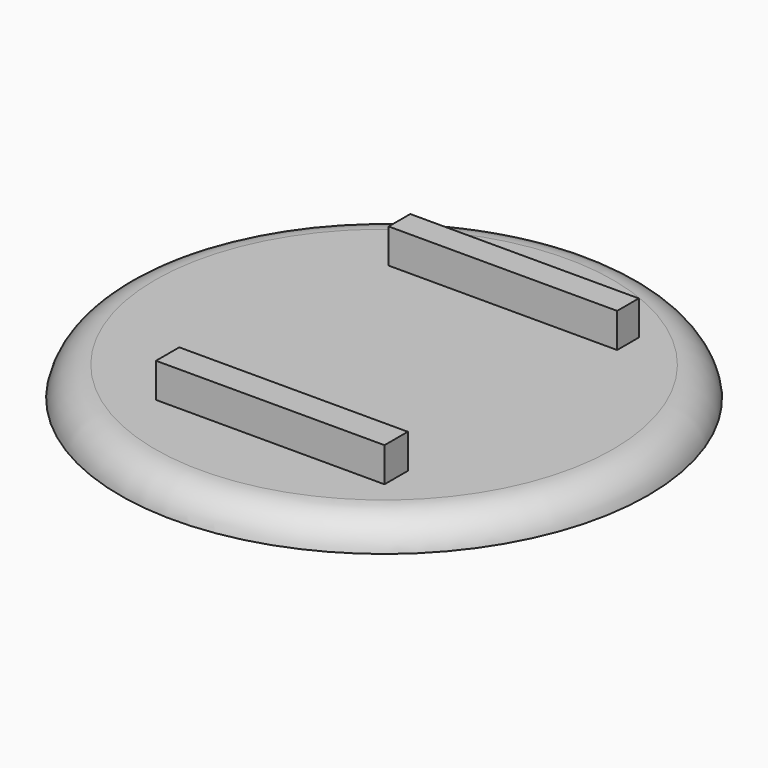
from build123d import *

# Parameters (mm, degrees)
F0_R     = 35.9935602645
F1_DEPTH = 4
F3_W     = 31.1600742862
F3_H     = 3.6825519055
F3_H_2   = 3.9658267051
F4_DEPTH = 4.7
F6_DEPTH = 2


# Not quite as in the source:
# - a fillet or chamfer that OpenCascade refuses, or shapes differently, is made with other operations: its cross-section is extruded or revolved along the edge and cut away or added


with BuildPart() as f1:
    # F0 (on Top) → F1 (new body)
    with BuildSketch(Plane.XY):
        Circle(F0_R)
    extrude(amount=F1_DEPTH)

    # F2: fillet of radius 4.8284271247 on 1 edges, made by hand

    # F2_s1 → F2_t2 (revolve, cut)
    with BuildSketch(Plane.XZ):
        with BuildLine():
            ThreePointArc((35.9935602645, 0), (34.3442797526, 2.8670910053), (31.2367318045, 4))
            Line((31.2367318045, 4), (35.9935602645, 4))
            Line((35.9935602645, 4), (35.9935602645, 0))
        make_face()
    revolve(axis=Axis((0, 0, 4), (0, 0, 1)), mode=Mode.SUBTRACT)

    # F3 (on face) → F4 (join)
    with BuildSketch(Plane.XY.offset(4)):
        with Locations((1.6996399499, 19.9707737193)):
            Rectangle(F3_W, F3_H)
        with Locations((1.6996399499, -19.5458633825)):
            Rectangle(F3_W, F3_H_2)
    extrude(amount=F4_DEPTH)

    # F5 (on face) → F6 (cut)
    with BuildSketch(Plane(origin=(0, 0, 0), x_dir=(1, 0, 0), z_dir=(0, 0, -1))):
        with BuildLine():
            Line((1.0116308873, -10.4608191177), (4.1609390889, -1.4550810977))
            ThreePointArc((4.1609390889, -1.4550810977), (-0.0142907136, -4.4080007801), (-4.1702862527, -1.4280713123))
            Line((-4.1702862527, -1.4280713123), (-1.0771154127, -10.4608191177))
            Line((-1.0771154127, -10.4608191177), (-1.0116308873, -10.4608191177))
            ThreePointArc((-1.0116308873, -10.4608191177), (0, -9.4491882305), (1.0116308873, -10.4608191177))
        make_face()
        with BuildLine():
            ThreePointArc((-1.0116308873, -10.4608191177), (0, -11.472450005), (1.0116308873, -10.4608191177))
            Line((1.0116308873, -10.4608191177), (0, -10.4608191177))
            Line((0, -10.4608191177), (-1.0116308873, -10.4608191177))
        make_face()
        with BuildLine():
            Line((0, -10.4608191177), (1.0116308873, -10.4608191177))
            ThreePointArc((1.0116308873, -10.4608191177), (0, -9.4491882305), (-1.0116308873, -10.4608191177))
            Line((-1.0116308873, -10.4608191177), (0, -10.4608191177))
        make_face()
        with BuildLine():
            ThreePointArc((4.1609390889, -1.4550810977), (4.3458137466, -0.7379552708), (4.4080239453, 0))
            ThreePointArc((4.4080239453, 0), (0.7238623632, 4.3481833426), (-4.1702862527, 1.4280713123))
            ThreePointArc((-4.1702862527, 1.4280713123), (-4.4080239453, 0), (-4.1702862527, -1.4280713123))
            ThreePointArc((-4.1702862527, -1.4280713123), (-0.0142907136, -4.4080007801), (4.1609390889, -1.4550810977))
        make_face()
        with BuildLine():
            ThreePointArc((-4.1702862527, 1.4280713123), (0.7238623632, 4.3481833426), (4.4080239453, 0))
            ThreePointArc((4.4080239453, 0), (4.3458137466, -0.7379552708), (4.1609390889, -1.4550810977))
            Line((4.1609390889, -1.4550810977), (4.6697812098, 0))
            Line((4.6697812098, 0), (1.0316451427, 10.5936024338))
            ThreePointArc((1.0316451427, 10.5936024338), (0, 9.5619572911), (-1.0316451427, 10.5936024338))
            Line((-1.0316451427, 10.5936024338), (-4.1702862527, 1.4280713123))
        make_face()
        with BuildLine():
            ThreePointArc((1.0316451427, 10.5936024338), (0, 11.6252475765), (-1.0316451427, 10.5936024338))
            Line((-1.0316451427, 10.5936024338), (0, 10.5936024338))
            Line((0, 10.5936024338), (1.0316451427, 10.5936024338))
        make_face()
        with BuildLine():
            Line((0, 10.5936024338), (-1.0316451427, 10.5936024338))
            ThreePointArc((-1.0316451427, 10.5936024338), (0, 9.5619572911), (1.0316451427, 10.5936024338))
            Line((1.0316451427, 10.5936024338), (0, 10.5936024338))
        make_face()
    extrude(amount=-F6_DEPTH, mode=Mode.SUBTRACT)


solid = f1.part
